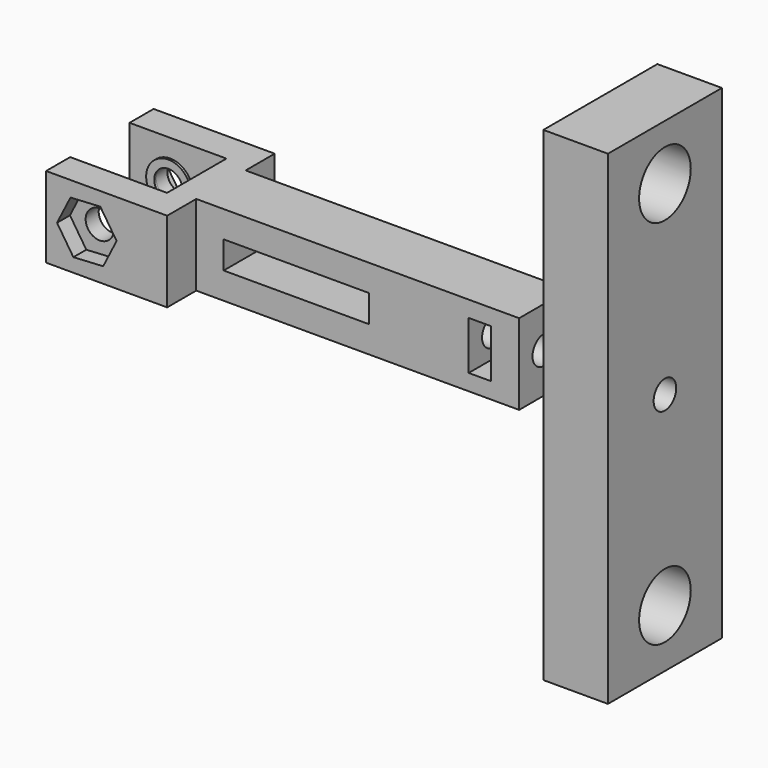
from build123d import *

# Parameters (mm, degrees)
F0_W      = 40
F0_H      = 3.825
F1_DEPTH  = 10
F2_R      = 1.75
F3_DEPTH  = 16.651
F4_W      = 18
F4_H      = 3.4
F4_W_2    = 2.75
F4_H_2    = 6
F5_DEPTH  = 12.151
F6_R      = 1.75
F7_DEPTH  = 15
F10_DEPTH = 2
F11_W     = 17.65
F11_H     = 60
F12_DEPTH = 8
F13_R     = 1.75
F14_DEPTH = 70.001
F15_R     = 2.75
F15_R_2   = 1.75
F16_DEPTH = 0.3
F17_R     = 1.75
F18_DEPTH = 2
F20_D     = 8


# Not quite as in the source:
# - a pattern or mirror of a feature is missing from the dataset's text; its kind, count and spacing are read off the source's solid


with BuildPart() as f1:
    # F0 (on Top) → F1 (new body)
    with BuildSketch(Plane.XY):
        Polygon((0, -3.825), (0, 0), (-3, 0), (-3, -4.6), (-15, -4.6), (-15, -8.325), (0, -8.325), align=None)
        Polygon((-3, 0), (0, 0), (0, 3.825), (0, 8.325), (-15, 8.325), (-15, 4.6), (-3, 4.6), align=None)
        with Locations((20, 1.9125)):
            Rectangle(F0_W, F0_H)
        with Locations((20, -1.9125)):
            Rectangle(F0_W, F0_H)
    extrude(amount=F1_DEPTH)

    # F2 (on face) → F3 (cut, through all)
    with BuildSketch(Plane.XZ.offset(8.325)):
        with Locations((-9.9527407438, 5)):
            Circle(F2_R)
    extrude(amount=-F3_DEPTH, mode=Mode.SUBTRACT)

    # F4 (on face) → F5 (cut, through all)
    with BuildSketch(Plane.XZ.offset(3.825)):
        with Locations((12.4002694301, 5)):
            Rectangle(F4_W, F4_H)
        with Locations((35.125, 5)):
            Rectangle(F4_W_2, F4_H_2)
    extrude(amount=-F5_DEPTH, mode=Mode.SUBTRACT)

    # F6 (on face) → F7 (cut)
    with BuildSketch(Plane.YZ.offset(40)):
        with Locations((0, 5)):
            Circle(F6_R)
    extrude(amount=-F7_DEPTH, mode=Mode.SUBTRACT)

    # F15 (on face) → F16 (join)
    with BuildSketch(Plane.XZ.offset(-4.6)):
        with Locations((-9.9527407438, 5)):
            Circle(F15_R)
        with Locations((-9.9527407438, 5)):
            Circle(F15_R_2, mode=Mode.SUBTRACT)
    f16 = extrude(amount=F16_DEPTH)

    # F16_copies: F16 across plane
    add(f16.mirror(Plane(origin=(0, 0, 0), x_dir=(0, 0, -1), z_dir=(0, -1, 0))))

    # F17 (on face) → F18 (cut)
    with BuildSketch(Plane.XZ.offset(8.325)):
        Polygon((-7.9284293953, 1.9088033227), (-6.2635302189, 5.2075067143), (-8.2878415673, 8.2987033916), (-11.9770520922, 8.0911966773), (-13.6419512686, 4.7924932857), (-11.6176399202, 1.7012966084), align=None)
        with Locations((-9.9527407438, 5)):
            Circle(F17_R, mode=Mode.SUBTRACT)
    f18 = extrude(amount=-F18_DEPTH, mode=Mode.SUBTRACT)

    # F18_copies: F18 across plane
    add(f18.mirror(Plane.ZX), mode=Mode.SUBTRACT)


with BuildPart() as f10:
    # F9 (on offset) → F10 (new body)
    with BuildSketch(Plane.YZ.offset(45)):
        Polygon((3.825, 0), (3.825, 10), (3.825, 19.8484882712), (-3.825, 19.8484882712), (-3.825, 10), (-3.825, 0), (-3.825, -10.1515117288), (3.825, -10.1515117288), align=None)
    extrude(amount=F10_DEPTH)

    # F11 (on face) → F12 (join)
    with BuildSketch(Plane.YZ.offset(47)):
        with Locations((0, 4.8484882712)):
            Rectangle(F11_W, F11_H)
    extrude(amount=F12_DEPTH)

    # F13 (on face) → F14 (cut, through all)
    with BuildSketch(Plane.YZ.offset(55)):
        with Locations((0, 5)):
            Circle(F13_R)
    extrude(amount=-F14_DEPTH, mode=Mode.SUBTRACT)

    # F20 (through all)
    with Locations(Plane(origin=(47, 0, 0), x_dir=(0, -1, 0), z_dir=(-1, 0, 0))):
        with Locations((0, -18), (0, 28)):
            Hole(F20_D / 2)


solid = Compound([f1.part, f10.part])
